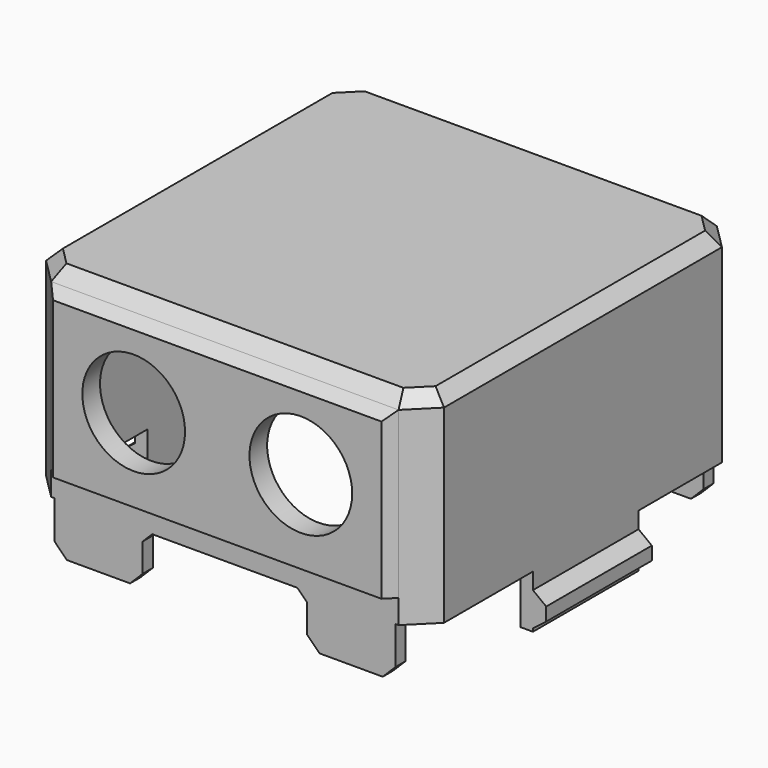
from build123d import *

# Parameters (mm, degrees)
F0_W      = 63
F0_H      = 63
F1_DEPTH  = 32
F2_SIZE   = 4
F3_SIZE   = 2
F4_T      = -2
F5_W      = 55
F5_H      = 26.2
F6_DEPTH  = 1.5
F7_SIZE   = 1.49999
F8_R      = 8.132
F9_DEPTH  = 3.5
F10_W     = 14
F10_H     = 8
F11_DEPTH = 2
F13_W     = 14
F13_H     = 8
F14_DEPTH = 2
F15_SIZE  = 2
F16_SIZE  = 1.5
F18_DEPTH = 9.9
F19_DEPTH = 11


# Not quite as in the source:
# - a fillet or chamfer is up to 0.001 mm smaller than in the source, because OpenCascade refuses the exact size
# - a pattern or mirror of a feature is missing from the dataset's text; its kind, count and spacing are read off the source's solid


with BuildPart() as f1:
    # F0 (on Top) → F1 (new body)
    with BuildSketch(Plane.XY):
        with Locations((31.5, 31.5)):
            Rectangle(F0_W, F0_H)
    extrude(amount=F1_DEPTH)

    # F2
    f2_edges = [f1.edges().sort_by_distance(p)[0] for p in [
        (63, 0, 16),
        (63, 63, 16),
        (0, 0, 16),
        (0, 63, 16),
    ]]
    chamfer(f2_edges, length=F2_SIZE)

    # F3
    f3_edges = [f1.edges().sort_by_distance(p)[0] for p in [
        (0, 31.5, 32),
        (2, 61, 32),
        (2, 2, 32),
        (31.5, 63, 32),
        (31.5, 0, 32),
        (61, 61, 32),
        (61, 2, 32),
        (63, 31.5, 32),
    ]]
    chamfer(f3_edges, length=F3_SIZE)

    # F4
    f4_openings = [f1.faces().sort_by_distance(p)[0] for p in [
        (31.5, 31.5, 0),
    ]]
    offset(amount=F4_T, openings=f4_openings)

    # F5 (on face) → F6 (join)
    with BuildSketch(Plane.XZ):
        with Locations((31.5, 16.9)):
            Rectangle(F5_W, F5_H)
    extrude(amount=F6_DEPTH)

    # F7 (size 1.5 in the source; OpenCascade refuses exactly that, so slightly less here)
    f7_edges = [f1.edges().sort_by_distance(p)[0] for p in [
        (31.5, -1.5, 30),
        (4, -1.5, 16.9),
        (59, -1.5, 16.9),
    ]]
    chamfer(f7_edges, length=F7_SIZE)

    # F8 (on face) → F9 (cut, through all)
    with BuildSketch(Plane.XZ.offset(1.5)):
        with Locations((18.269, 16.955)):
            Circle(F8_R)
        with Locations((44.731, 16.955)):
            Circle(F8_R)
    extrude(amount=-F9_DEPTH, mode=Mode.SUBTRACT)

    # F10 (on face) → F11 (join, through all)
    with BuildSketch(Plane.XZ):
        with Locations((11.5, -4)):
            Rectangle(F10_W, F10_H)
        with Locations((51.5, -4)):
            Rectangle(F10_W, F10_H)
    extrude(amount=-F11_DEPTH)

    # F13 (on face) → F14 (join)
    with BuildSketch(Plane(origin=(0, 63, 0), x_dir=(-1, 0, 0), z_dir=(0, 1, 0))):
        with Locations((-51.5, -4)):
            Rectangle(F13_W, F13_H)
        with Locations((-11.5, -4)):
            Rectangle(F13_W, F13_H)
    extrude(amount=-F14_DEPTH)

    # F15
    f15_edges = [f1.edges().sort_by_distance(p)[0] for p in [
        (4.5, 1, -8),
        (18.5, 1, -8),
        (44.5, 1, -8),
        (58.5, 1, -8),
        (18.5, 62, -8),
        (4.5, 62, -8),
        (58.5, 62, -8),
        (44.5, 62, -8),
    ]]
    chamfer(f15_edges, length=F15_SIZE)

    # F16
    f16_edges = [f1.edges().sort_by_distance(p)[0] for p in [
        (18.5, 62, 0),
        (18.5, 1, 0),
        (44.5, 1, 0),
        (44.5, 62, 0),
    ]]
    chamfer(f16_edges, length=F16_SIZE)

    # F17 (on mid) → F18 (join)
    with BuildSketch(Plane(origin=(0, 31.5, 0), x_dir=(-1, 0, 0), z_dir=(0, 1, 0))):
        Polygon((0, -2.6), (0, 0), (-2, 0), (-2, -8.4), (0, -8.4), (0, -7.9), align=None)
        Polygon((2.1, -4.2), (0, -2.6), (0, -7.9), (2.1, -6.3), align=None)
    f18 = extrude(amount=-F18_DEPTH)

    # F18_copies: F18 across plane
    add(f18.mirror(Plane(origin=(31.5, 0, 0), x_dir=(0, 0, 1), z_dir=(1, 0, 0))))

    # F19 (add): a face of the model
    f19_faces = [f1.faces().sort_by_distance(p)[0] for p in [
        (0.3995726496, 31.5, -4.5320512821),
    ]]
    f19 = extrude(f19_faces, amount=F19_DEPTH)

    # F19_copies: F19 across plane
    add(f19.mirror(Plane(origin=(31.5, 0, 0), x_dir=(0, 0, 1), z_dir=(1, 0, 0))))


solid = f1.part
